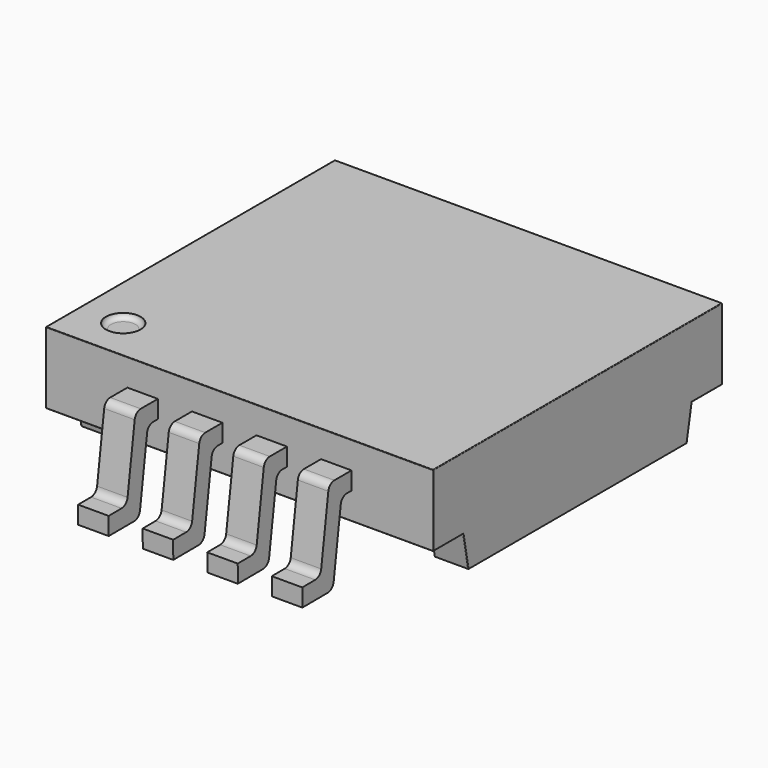
from build123d import *

# Parameters (mm, degrees)
F0_W     = 7.62
F0_H     = 7.11
F1_DEPTH = 0.705
F3_DEPTH = 0.66
F5_DEPTH = 25
F6_R     = 0.01
F7_R     = 0.3408088795
F8_DEPTH = 0.1
F9_R     = 0.09999
F11_W    = 0.6
F11_H    = 0.35
F13_R    = 0.1
F14_W    = 0.6
F14_H    = 0.3504652178
F16_R    = 0.15


# Not quite as in the source:
# - a fillet or chamfer is up to 0.001 mm smaller than in the source, because OpenCascade refuses the exact size
# - a feature names something its author has since deleted; it is built from what else it names


with BuildPart() as f1:
    # F0 (on Top) → F1 (new body, symmetric)
    with BuildSketch(Plane.XY):
        Rectangle(F0_W, F0_H)
    extrude(amount=F1_DEPTH, both=True)

    # F2 (on face) → F3 (join)
    with BuildSketch(Plane(origin=(0, 0, -0.705), x_dir=(1, 0, 0), z_dir=(0, 0, -1))):
        Polygon((-3.81, 2.81), (-3.81, 0), (-3.81, -2.81), (-3.15, -2.81), (-3.15, 2.81), align=None)
        Polygon((3.81, 0), (3.81, 2.81), (3.15, 2.81), (3.15, -2.81), (3.81, -2.81), align=None)
    extrude(amount=F3_DEPTH)

    # F4 (on face) → F5 (cut)
    with BuildSketch(Plane(origin=(-3.81, 0, 0), x_dir=(0, -1, 0), z_dir=(-1, 0, 0))):
        Polygon((-2.81, -1.365), (-2.6863825042, -1.365), (-2.81, -0.705), align=None)
        Polygon((2.81, -1.365), (2.81, -0.705), (2.6863825042, -1.365), align=None)
    extrude(amount=-F5_DEPTH, mode=Mode.SUBTRACT)

    # F6
    f6_edges = [f1.edges().sort_by_distance(p)[0] for p in [
        (-3.81, 0, 0.705),
        (-3.81, -3.555, 0),
        (0, -3.555, 0.705),
        (-3.81, 3.555, 0),
        (3.81, -3.555, 0),
        (3.81, 0, 0.705),
        (3.81, 3.555, 0),
        (0, 3.555, 0.705),
        (0, 3.555, -0.705),
        (0, -3.555, -0.705),
        (3.81, -3.1825, -0.705),
        (3.81, -2.748191, -1.035),
        (3.81, 2.748191, -1.035),
        (3.81, 3.1825, -0.705),
        (-3.81, -2.748191, -1.035),
        (-3.81, -3.1825, -0.705),
        (-3.81, 3.1825, -0.705),
        (-3.81, 2.748191, -1.035),
    ]]
    fillet(f6_edges, radius=F6_R)

    # F7 (on face) → F8 (cut)
    with BuildSketch(Plane.XY.offset(0.705)):
        with Locations((-2.9591911205, -2.7141911205)):
            Circle(F7_R)
    extrude(amount=-F8_DEPTH, mode=Mode.SUBTRACT)

    # F9 (radius 0.1 in the source; OpenCascade refuses exactly that, so slightly less here)
    f9_edges = [f1.edges().sort_by_distance(p)[0] for p in [
        (-3.3, -2.714191, 0.605),
    ]]
    fillet(f9_edges, radius=F9_R)

    # F12: sweep along a path in F10
    with BuildLine(Plane.YZ) as f12_path:
        Line((3.555, 0), (3.955, 0))
        Line((3.955, 0), (4.165, -1.5318583786))
        Line((4.165, -1.5318583786), (4.765, -1.535))
    # F11 (on face) → F12 (sweep)
    with BuildSketch(Plane(origin=(0, 3.555, 0), x_dir=(-1, 0, 0), z_dir=(0, 1, 0))):
        with Locations((-1.905, 0)):
            Rectangle(F11_W, F11_H)
        with Locations((-0.635, 0)):
            Rectangle(F11_W, F11_H)
        with Locations((0.635, 0)):
            Rectangle(F11_W, F11_H)
        with Locations((1.905, 0)):
            Rectangle(F11_W, F11_H)
    sweep(path=f12_path.line, transition=Transition.RIGHT)

    # F13
    f13_edges = [f1.edges().sort_by_distance(p)[0] for p in [
        (-1.905, 4.107646, 0.175),
        (-1.905, 4.317756, -1.357656),
        (-0.635, 4.107646, 0.175),
        (-0.635, 4.317756, -1.357656),
        (0.635, 4.107646, 0.175),
        (0.635, 4.317756, -1.357656),
        (1.905, 4.107646, 0.175),
        (1.905, 4.317756, -1.357656),
        (1.905, 3.802354, -0.175),
        (0.635, 3.802354, -0.175),
        (-0.635, 3.802354, -0.175),
        (-1.905, 3.802354, -0.175),
        (-1.905, 4.012244, -1.706061),
        (-0.635, 4.012244, -1.706061),
        (0.635, 4.012244, -1.706061),
        (1.905, 4.012244, -1.706061),
    ]]
    fillet(f13_edges, radius=F13_R)

    # F15: sweep along a path in F10
    with BuildLine(Plane.YZ) as f15_path:
        Line((-3.555, 0), (-3.955, 0))
        Line((-3.955, 0), (-4.165, -1.5318583786))
        Line((-4.165, -1.5318583786), (-4.765, -1.535))
    # F14 (on face) → F15 (sweep)
    with BuildSketch(Plane.XZ.offset(3.555)):
        with Locations((-1.905, 0)):
            Rectangle(F14_W, F14_H)
        with Locations((-0.635, 0)):
            Rectangle(F14_W, F14_H)
        with Locations((0.635, 0)):
            Rectangle(F14_W, F14_H)
        with Locations((1.905, 0)):
            Rectangle(F14_W, F14_H)
    sweep(path=f15_path.line, transition=Transition.RIGHT)

    # F16
    f16_edges = [f1.edges().sort_by_distance(p)[0] for p in [
        (-1.905, -4.107849, 0.175233),
        (-0.635, -4.107849, 0.175233),
        (0.635, -4.107849, 0.175233),
        (1.905, -4.107849, 0.175233),
        (-1.905, -4.317959, -1.357424),
        (-0.635, -4.317959, -1.357424),
        (0.635, -4.317959, -1.357424),
        (1.905, -4.317959, -1.357424),
        (-1.905, -3.802151, -0.175233),
        (-0.635, -3.802151, -0.175233),
        (0.635, -3.802151, -0.175233),
        (1.905, -3.802151, -0.175233),
        (0.635, -4.012041, -1.706292),
        (-0.635, -4.012041, -1.706292),
        (-1.905, -4.012041, -1.706292),
        (1.905, -4.012041, -1.706292),
    ]]
    fillet(f16_edges, radius=F16_R)


solid = f1.part
